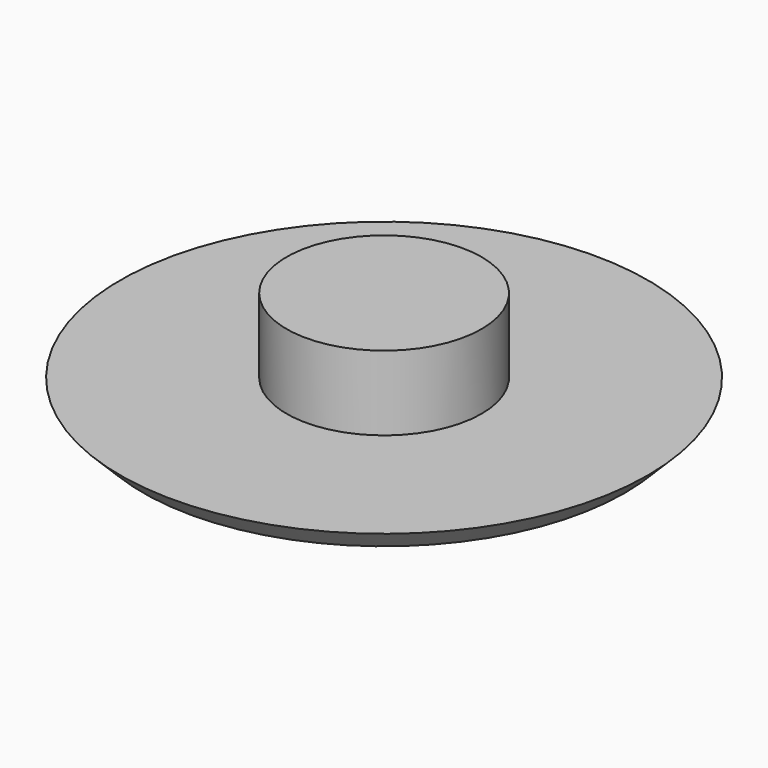
from build123d import *

# Parameters (mm, degrees)
F0_R     = 11.5
F1_DEPTH = 1
F2_R     = 4.25
F3_DEPTH = 3.25
F4_SIZE  = 0.99999


# Not quite as in the source:
# - a fillet or chamfer is up to 0.001 mm smaller than in the source, because OpenCascade refuses the exact size


with BuildPart() as f1:
    # F0 (on Top) → F1 (new body)
    with BuildSketch(Plane.XY):
        Circle(F0_R)
    extrude(amount=F1_DEPTH)

    # F2 (on face) → F3 (join)
    with BuildSketch(Plane.XY.offset(1)):
        Circle(F2_R)
    extrude(amount=F3_DEPTH)

    # F4 (size 1 in the source; OpenCascade refuses exactly that, so slightly less here)
    f4_edges = [f1.edges().sort_by_distance(p)[0] for p in [
        (-11.5, 0, 0),
    ]]
    chamfer(f4_edges, length=F4_SIZE)


solid = f1.part
